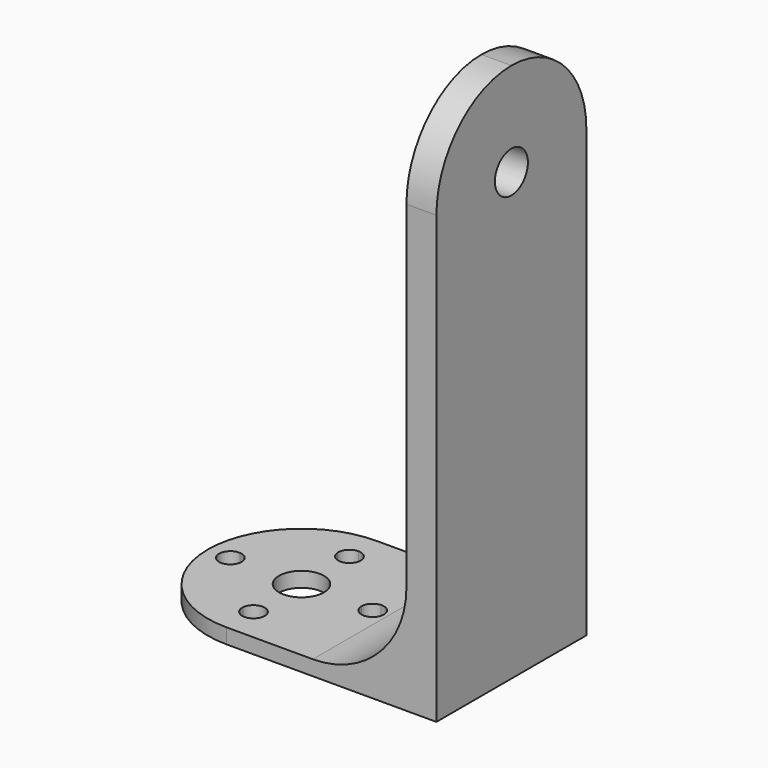
from build123d import *

# Parameters (mm, degrees)
F0_R     = 3
F1_DEPTH = 2
F2_W     = 4
F2_H     = 25
F3_DEPTH = 70
F4_R     = 2.75
F5_DEPTH = 40.501
F6_R     = 12.49999


# Not quite as in the source:
# - a fillet or chamfer is up to 0.001 mm smaller than in the source, because OpenCascade refuses the exact size


with BuildPart() as f1:
    # F0 (on Top) → F1 (new body)
    with BuildSketch(Plane.XY):
        with BuildLine():
            ThreePointArc((0, -12.5), (8.8388347648, -8.8388347648), (12.5, 0))
            ThreePointArc((12.5, 0), (8.8388347648, 8.8388347648), (0, 12.5))
            ThreePointArc((0, 12.5), (-12.5, 0), (0, -12.5))
        make_face()
        with BuildLine():
            ThreePointArc((0, 9.5), (6.1662175321, 7.2268777039), (9.3815789474, 1.4953181783))
            ThreePointArc((9.3815789474, 1.4953181783), (10.5179313388, 1.1017330845), (11, 0))
            ThreePointArc((11, 0), (10.5179313388, -1.1017330845), (9.3815789474, -1.4953181783))
            ThreePointArc((9.3815789474, -1.4953181783), (6.1662175364, -7.2268777002), (1.13e-08, -9.5))
            ThreePointArc((1.13e-08, -9.5), (-6.1662175278, -7.2268777076), (-9.3815789474, -1.4953181783))
            ThreePointArc((-9.3815789474, -1.4953181783), (-11, 0), (-9.3815789474, 1.4953181783))
            ThreePointArc((-9.3815789474, 1.4953181783), (-6.1662175321, 7.2268777039), (0, 9.5))
        make_face(mode=Mode.SUBTRACT)
        with BuildLine():
            ThreePointArc((1.4933936552, -7.859375), (6.1622702489, -5.1016100771), (8, 0))
            ThreePointArc((8, 0), (6.1622702489, 5.1016100771), (1.4933936552, 7.859375))
            ThreePointArc((1.4933936552, 7.859375), (0, 6.5), (-1.4933936552, 7.859375))
            ThreePointArc((-1.4933936552, 7.859375), (-6.1622702489, 5.1016100771), (-8, 0))
            ThreePointArc((-8, 0), (-6.1622702489, -5.1016100771), (-1.4933936552, -7.859375))
            ThreePointArc((-1.4933936552, -7.859375), (0, -6.5), (1.4933936552, -7.859375))
        make_face()
        Circle(F0_R, mode=Mode.SUBTRACT)
        with BuildLine():
            ThreePointArc((0, 12.5), (8.8388347648, 8.8388347648), (12.5, 0))
            ThreePointArc((12.5, 0), (8.8388347648, -8.8388347648), (0, -12.5))
            Line((0, -12.5), (28, -12.5))
            Line((28, -12.5), (28, 12.5))
            Line((28, 12.5), (0, 12.5))
        make_face()
        with BuildLine():
            ThreePointArc((-1.4933936552, 7.859375), (-1.1092649593, 9.0097184013), (0, 9.5))
            ThreePointArc((0, 9.5), (-6.1662175321, 7.2268777039), (-9.3815789474, 1.4953181783))
            ThreePointArc((-9.3815789474, 1.4953181783), (-8.3982669155, 1.0179313388), (-8, 0))
            ThreePointArc((-8, 0), (-6.1622702489, 5.1016100771), (-1.4933936552, 7.859375))
        make_face()
        with BuildLine():
            ThreePointArc((8, 0), (8.3982669155, 1.0179313388), (9.3815789474, 1.4953181783))
            ThreePointArc((9.3815789474, 1.4953181783), (6.1662175321, 7.2268777039), (0, 9.5))
            ThreePointArc((0, 9.5), (1.0606601718, 9.0606601718), (1.5, 8))
            ThreePointArc((1.5, 8), (1.4983475036, 7.9296099538), (1.4933936552, 7.859375))
            ThreePointArc((1.4933936552, 7.859375), (6.1622702489, 5.1016100771), (8, 0))
        make_face()
        with BuildLine():
            ThreePointArc((1.13e-08, -9.5), (6.1662175364, -7.2268777002), (9.3815789474, -1.4953181783))
            ThreePointArc((9.3815789474, -1.4953181783), (8.3982669155, -1.0179313388), (8, 0))
            ThreePointArc((8, 0), (6.1622702489, -5.1016100771), (1.4933936552, -7.859375))
            ThreePointArc((1.4933936552, -7.859375), (1.4983475036, -7.9296099538), (1.5, -8))
            ThreePointArc((1.5, -8), (1.0606601758, -9.0606601678), (1.13e-08, -9.5))
        make_face()
        with BuildLine():
            ThreePointArc((-9.3815789474, -1.4953181783), (-6.1662175278, -7.2268777076), (1.13e-08, -9.5))
            ThreePointArc((1.13e-08, -9.5), (-1.1092649555, -9.0097184055), (-1.4933936552, -7.859375))
            ThreePointArc((-1.4933936552, -7.859375), (-6.1622702489, -5.1016100771), (-8, 0))
            ThreePointArc((-8, 0), (-8.3982669155, -1.0179313388), (-9.3815789474, -1.4953181783))
        make_face()
    extrude(amount=F1_DEPTH)

    # F2 (on face) → F3 (join)
    with BuildSketch(Plane.XY.offset(2)):
        with Locations((26, 0)):
            Rectangle(F2_W, F2_H)
    extrude(amount=F3_DEPTH)

    # F4 (on face) → F5 (cut, through all)
    with BuildSketch(Plane.YZ.offset(28)):
        with Locations((0, 59.5)):
            Circle(F4_R)
    extrude(amount=-F5_DEPTH, mode=Mode.SUBTRACT)

    # F6 (radius 12.5 in the source; OpenCascade refuses exactly that, so slightly less here)
    f6_edges = [f1.edges().sort_by_distance(p)[0] for p in [
        (24, 0, 2),
        (26, -12.5, 72),
        (26, 12.5, 72),
    ]]
    fillet(f6_edges, radius=F6_R)


solid = f1.part
